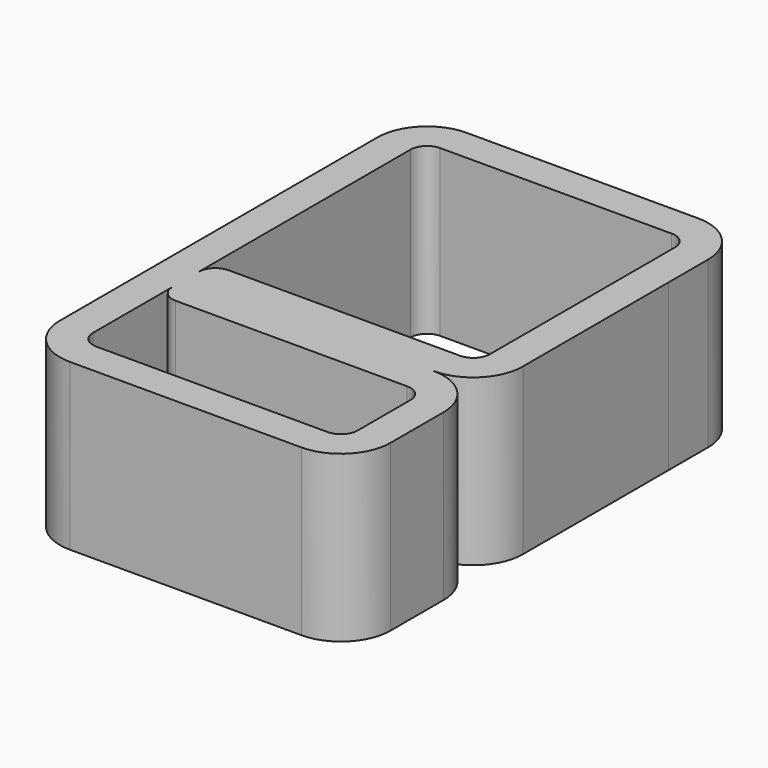
from build123d import *

# Parameters (mm, degrees)
F1_DEPTH = 15.875


# Not quite as in the source:
# - ends of sketch curves that miss each other by under 0.0002 mm in the source are joined
# - the program builds the solid bodies; features that only make, move or delete a surface that nothing else refers to are left out


with BuildPart() as f1:
    # F0 (on Top) → F1 (new body)
    with BuildSketch(Plane.XY):
        with BuildLine():
            Line((-11.1125005688, -19.05), (11.1124994312, -19.05))
            ThreePointArc((11.1124994312, -19.05), (14.4800954095, -17.6550961124), (15.8749994312, -14.2875001896))
            Line((15.8749994312, -14.2875001896), (15.874999684, -7.9375001896))
            ThreePointArc((15.874999684, -7.9375001896), (14.4800957964, -4.5699040216), (11.112499684, -3.175))
            ThreePointArc((11.112499684, -3.175), (14.4800960416, -1.7800961124), (15.8750000632, 1.5874998104))
            Line((15.8750000632, 1.5874998104), (15.8750007584, 19.05))
            Line((15.8750007584, 19.05), (15.8750007584, 23.8125))
            ThreePointArc((15.8750007584, 23.8125), (14.4800968038, 27.1800960454), (11.1125007584, 28.575))
            Line((11.1125007584, 28.575), (-11.1124992416, 28.575))
            ThreePointArc((-11.1124992416, 28.575), (-14.480095287, 27.1800960454), (-15.8749992416, 23.8125))
            Line((-15.8749992416, 23.8125), (-15.8749992416, 19.05))
            Line((-15.8749992416, 19.05), (-15.8750005688, -14.2874998104))
            ThreePointArc((-15.8750005688, -14.2874998104), (-14.4800966813, -17.6550959784), (-11.1125005688, -19.05))
        make_face()
        with BuildLine():
            Line((-12.7, -6.35), (-12.7, -4.7625))
            ThreePointArc((-12.7, -4.7625), (-12.2350320151, -5.8850320151), (-11.1125, -6.35))
            Line((-11.1125, -6.35), (11.1125, -6.35))
            ThreePointArc((11.1125, -6.35), (12.2350320151, -6.8149679849), (12.7, -7.9375))
            Line((12.7, -7.9375), (12.7, -14.2875))
            ThreePointArc((12.7, -14.2875), (12.2350320151, -15.4100320151), (11.1125, -15.875))
            Line((11.1125, -15.875), (-11.1125, -15.875))
            ThreePointArc((-11.1125, -15.875), (-12.2350320151, -15.4100320151), (-12.7, -14.2875))
            Line((-12.7, -14.2875), (-12.7, -6.35))
        make_face(mode=Mode.SUBTRACT)
        with BuildLine():
            ThreePointArc((-12.7, -1.5875), (-12.2350320151, -2.7100320151), (-11.1125, -3.175))
            ThreePointArc((-11.1125, -3.175), (-12.2350320151, -3.6399679849), (-12.7, -4.7625))
            Line((-12.7, -4.7625), (-12.7, -3.175))
            Line((-12.7, -3.175), (-12.7, -1.5875))
        make_face(mode=Mode.SUBTRACT)
        with BuildLine():
            ThreePointArc((-11.1125, 0), (-12.2350320151, -0.4649679849), (-12.7, -1.5875))
            Line((-12.7, -1.5875), (-12.7, 0))
            Line((-12.7, 0), (-12.7, 23.8125))
            ThreePointArc((-12.7, 23.8125), (-12.2350320151, 24.9350320151), (-11.1125, 25.4))
            Line((-11.1125, 25.4), (11.1125, 25.4))
            ThreePointArc((11.1125, 25.4), (12.2350320151, 24.9350320151), (12.7, 23.8125))
            Line((12.7, 23.8125), (12.7, 1.5875))
            ThreePointArc((12.7, 1.5875), (12.2350320151, 0.4649679849), (11.1125, 0))
            Line((11.1125, 0), (-11.1125, 0))
        make_face(mode=Mode.SUBTRACT)
        with BuildLine():
            Line((-12.7, -3.175), (-11.1125, -3.175))
            ThreePointArc((-11.1125, -3.175), (-12.2350320151, -2.7100320151), (-12.7, -1.5875))
            Line((-12.7, -1.5875), (-12.7, -3.175))
        make_face()
        with BuildLine():
            ThreePointArc((-12.7, -4.7625), (-12.2350320151, -3.6399679849), (-11.1125, -3.175))
            Line((-11.1125, -3.175), (-12.7, -3.175))
            Line((-12.7, -3.175), (-12.7, -4.7625))
        make_face()
    extrude(amount=F1_DEPTH)


solid = f1.part
